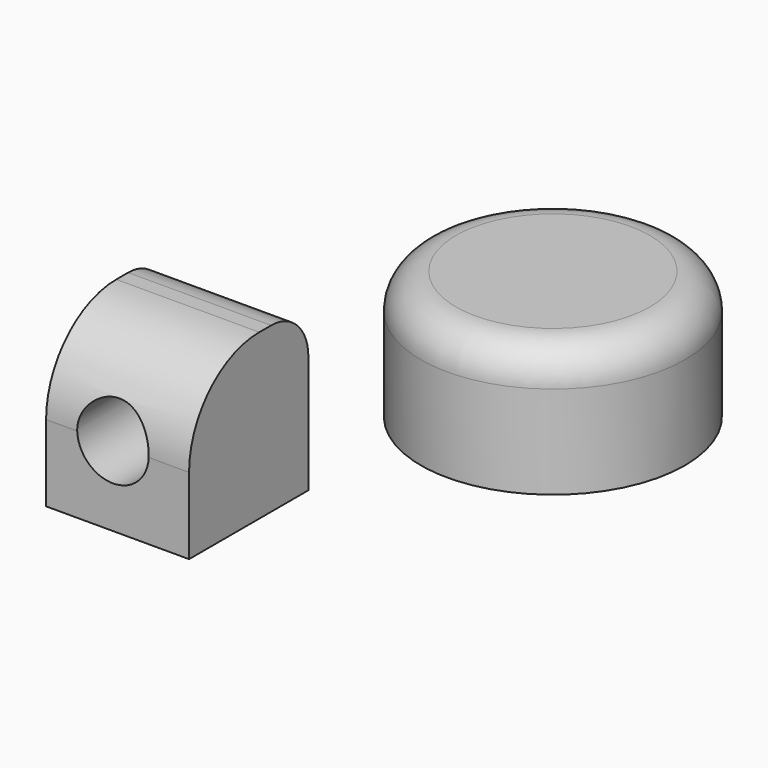
from build123d import *

# Parameters (mm, degrees)
F0_R        = 75.2432025663
F1_DEPTH    = 73
F2_W        = 81.4927220345
F2_H        = 93.5291722417
F2_R        = 20.3787621881
F3_DEPTH    = 85
F4_T1_DEPTH = 331.4927220345
F5_R        = 26.5563491861
F6_R        = 20


# Not quite as in the source:
# - a fillet or chamfer that OpenCascade refuses, or shapes differently, is made with other operations: its cross-section is extruded or revolved along the edge and cut away or added


with BuildPart() as f1:
    # F0 (on Top) → F1 (new body)
    with BuildSketch(Plane.XY):
        Circle(F0_R)
    extrude(amount=F1_DEPTH)

    # F6
    f6_edges = [f1.edges().sort_by_distance(p)[0] for p in [
        (-75.243203, 0, 73),
    ]]
    fillet(f6_edges, radius=F6_R)


with BuildPart() as f3:
    # F2 (on Front) → F3 (new body)
    with BuildSketch(Plane.XZ):
        with Locations((-180.1057755947, -35.4908742011)):
            Rectangle(F2_W, F2_H)
        with Locations((-182.736903429, -37.9713438451)):
            Circle(F2_R, mode=Mode.SUBTRACT)
    extrude(amount=F3_DEPTH)

    # F4: fillet of radius 50 on 1 edges, made by hand

    # F4_s2 → F4_t1 (cut)
    with BuildSketch(Plane.YZ.offset(-345.8521366119)):
        with BuildLine():
            ThreePointArc((-35, 11.2737119198), (-70.3553390593, -3.3709490209), (-85, -38.7262880802))
            Line((-85, -38.7262880802), (-85, 11.2737119198))
            Line((-85, 11.2737119198), (-35, 11.2737119198))
        make_face()
    extrude(amount=F4_T1_DEPTH, mode=Mode.SUBTRACT)

    # F5
    f5_edges = [f3.edges().sort_by_distance(p)[0] for p in [
        (-180.105776, 0, 11.273712),
    ]]
    fillet(f5_edges, radius=F5_R)


solid = Compound([f1.part, f3.part])
